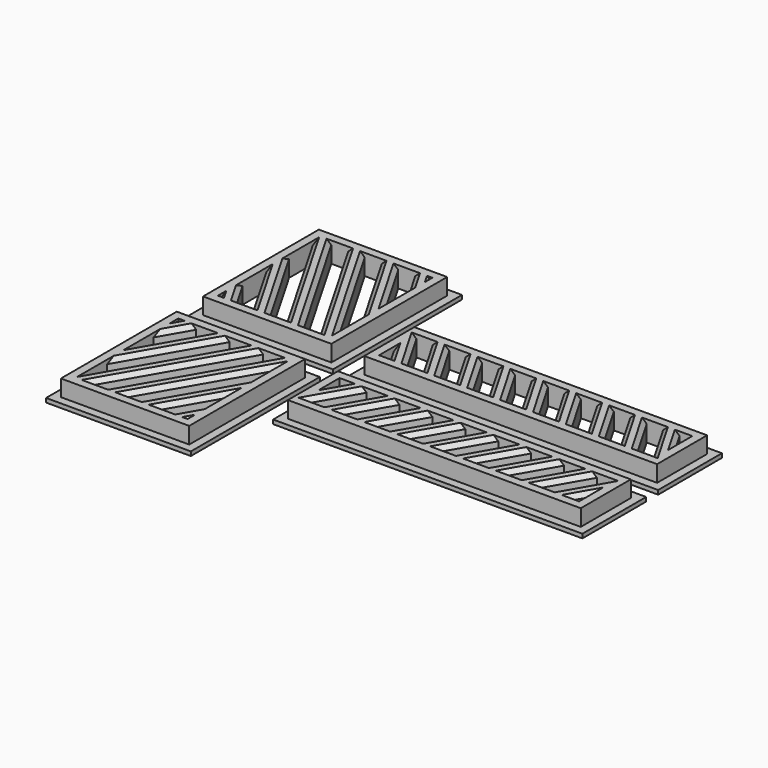
from build123d import *

# Parameters (mm, degrees)
F0_W      = 15.6
F0_H      = 17.6
F1_DEPTH  = 2.5
F2_W      = 35.7645684853
F2_H      = 21.2578142527
F3_DEPTH  = 10
F4_W      = 15.6
F4_H      = 17.6
F4_W_2    = 13.6
F4_H_2    = 15.6
F5_DEPTH  = 2.5
F6_W      = 17.6
F6_H      = 19.6
F6_W_2    = 15.6
F6_H_2    = 17.6
F7_DEPTH  = 0.5
F8_SIZE   = 0.5
F9_W      = 35.6
F9_H      = 7.6
F10_DEPTH = 2.5
F11_W     = 70.1136225462
F11_H     = 15.9944170155
F12_DEPTH = 25
F13_W     = 35.6
F13_H     = 7.6
F13_W_2   = 33.6
F13_H_2   = 5.6
F14_DEPTH = 2.5
F15_W     = 37.6
F15_H     = 9.6891392594
F15_W_2   = 35.6
F15_H_2   = 7.6
F16_DEPTH = 0.5
F17_SIZE  = 0.5


with BuildPart() as f1:
    # F0 (on Top) → F1 (new body)
    with BuildSketch(Plane.XY):
        with Locations((-9.8, 8.8)):
            Rectangle(F0_W, F0_H)
    extrude(amount=F1_DEPTH)

    # F2 (on Top) → F3 (cut)
    with BuildSketch(Plane.XY):
        with Locations((-9.857636116, 8.6271929322)):
            Rectangle(F2_W, F2_H)
        Polygon((-13.85, 0), (-15.85, 0), (-26.0113647377, 17.6), (-24.0113647377, 17.6), align=None, mode=Mode.SUBTRACT)
        Polygon((-21.940212315, 17.6), (-19.940212315, 17.6), (-9.7788475773, 0), (-11.7788475773, 0), align=None, mode=Mode.SUBTRACT)
        Polygon((-17.8690598923, 17.6), (-15.8690598923, 17.6), (-5.7076951546, 0), (-7.7076951546, 0), align=None, mode=Mode.SUBTRACT)
        Polygon((-13.7979074696, 17.6), (-11.7979074696, 17.6), (-1.6365427319, 0), (-3.6365427319, 0), align=None, mode=Mode.SUBTRACT)
        Polygon((-9.7267550469, 17.6), (-7.7267550469, 17.6), (2.4346096908, 0), (0.4346096908, 0), align=None, mode=Mode.SUBTRACT)
        Polygon((-5.6556026242, 17.6), (-3.6556026242, 17.6), (6.5057621135, 0), (4.5057621135, 0), align=None, mode=Mode.SUBTRACT)
    extrude(amount=F3_DEPTH, mode=Mode.SUBTRACT)

    # F4 (on Top) → F5 (join)
    with BuildSketch(Plane.XY):
        with Locations((-9.8, 8.8)):
            Rectangle(F4_W, F4_H)
        with Locations((-9.8, 8.8)):
            Rectangle(F4_W_2, F4_H_2, mode=Mode.SUBTRACT)
    extrude(amount=F5_DEPTH)

    # F6 (on face) → F7 (join)
    with BuildSketch(Plane(origin=(0, 0, 0), x_dir=(1, 0, 0), z_dir=(0, 0, -1))):
        with Locations((-9.8, -8.8)):
            Rectangle(F6_W, F6_H)
        with Locations((-9.8, -8.8)):
            Rectangle(F6_W_2, F6_H_2, mode=Mode.SUBTRACT)
    extrude(amount=-F7_DEPTH)

    # F8
    f8_edges = [f1.edges().sort_by_distance(p)[0] for p in [
        (-15.513675, 2.88157, 2.5),
        (-14.478099, 4.67524, 2.5),
        (-12.442523, 8.200962, 0),
        (-10.788378, 8.8, 2.5),
        (-8.717225, 8.8, 2.5),
        (-7.110279, 9.480789, 2.5),
        (-6.074702, 11.274459, 2.5),
        (-5.074702, 13.00651, 2.5),
        (-4.039126, 14.800181, 2.5),
        (-16.513675, 1.149519, 2.5),
        (-3.039126, 16.532231, 2.5),
        (-12.442523, 8.200962, 2.5),
        (-13.478099, 6.407291, 2.5),
    ]]
    chamfer(f8_edges, length=F8_SIZE)


with BuildPart() as f10:
    # F9 (on Top) → F10 (new body)
    with BuildSketch(Plane.XY):
        with Locations((19.8, 3.8)):
            Rectangle(F9_W, F9_H)
    extrude(amount=F10_DEPTH)

    # F11 (on Top) → F12 (cut)
    with BuildSketch(Plane.XY):
        with Locations((32.6393267076, 4.0027914923)):
            Rectangle(F11_W, F11_H)
        Polygon((6.8688021535, 0), (4.8688021535, 0), (0.25, 8), (2.25, 8), align=None, mode=Mode.SUBTRACT)
        Polygon((6.25, 8), (10.8688021535, 0), (8.8688021535, 0), (4.25, 8), align=None, mode=Mode.SUBTRACT)
        Polygon((10.25, 8), (14.8688021535, 0), (12.8688021535, 0), (8.25, 8), align=None, mode=Mode.SUBTRACT)
        Polygon((14.25, 8), (18.8688021535, 0), (16.8688021535, 0), (12.25, 8), align=None, mode=Mode.SUBTRACT)
        Polygon((18.25, 8), (22.8688021535, 0), (20.8688021535, 0), (16.25, 8), align=None, mode=Mode.SUBTRACT)
        Polygon((22.25, 8), (26.8688021535, 0), (24.8688021535, 0), (20.25, 8), align=None, mode=Mode.SUBTRACT)
        Polygon((26.25, 8), (30.8688021535, 0), (28.8688021535, 0), (24.25, 8), align=None, mode=Mode.SUBTRACT)
        Polygon((30.25, 8), (34.8688021535, 0), (32.8688021535, 0), (28.25, 8), align=None, mode=Mode.SUBTRACT)
        Polygon((34.25, 8), (38.8688021535, 0), (36.8688021535, 0), (32.25, 8), align=None, mode=Mode.SUBTRACT)
        Polygon((38.25, 8), (42.8688021535, 0), (40.8688021535, 0), (36.25, 8), align=None, mode=Mode.SUBTRACT)
        Polygon((42.25, 8), (46.8688021535, 0), (44.8688021535, 0), (40.25, 8), align=None, mode=Mode.SUBTRACT)
        Polygon((46.25, 8), (50.8688021535, 0), (48.8688021535, 0), (44.25, 8), align=None, mode=Mode.SUBTRACT)
        Polygon((50.25, 8), (54.8688021535, 0), (52.8688021535, 0), (48.25, 8), align=None, mode=Mode.SUBTRACT)
        Polygon((54.25, 8), (58.8688021535, 0), (56.8688021535, 0), (52.25, 8), align=None, mode=Mode.SUBTRACT)
        Polygon((58.25, 8), (62.8688021535, 0), (60.8688021535, 0), (56.25, 8), align=None, mode=Mode.SUBTRACT)
    extrude(amount=F12_DEPTH, mode=Mode.SUBTRACT)

    # F13 (on Top) → F14 (join)
    with BuildSketch(Plane.XY):
        with Locations((19.8, 3.8)):
            Rectangle(F13_W, F13_H)
        with Locations((19.8, 3.8)):
            Rectangle(F13_W_2, F13_H_2, mode=Mode.SUBTRACT)
    extrude(amount=F14_DEPTH)

    # F15 (on face) → F16 (join)
    with BuildSketch(Plane(origin=(0, 0, 0), x_dir=(1, 0, 0), z_dir=(0, 0, -1))):
        with Locations((19.8, -3.7554303703)):
            Rectangle(F15_W, F15_H)
        with Locations((19.8, -3.8)):
            Rectangle(F15_W_2, F15_H_2, mode=Mode.SUBTRACT)
    extrude(amount=-F16_DEPTH)

    # F17
    f17_edges = [f10.edges().sort_by_distance(p)[0] for p in [
        (8.674871, 3.8, 2.5),
        (10.674871, 3.8, 2.5),
        (12.674871, 3.8, 2.5),
        (14.674871, 3.8, 2.5),
        (16.674871, 3.8, 2.5),
        (18.674871, 3.8, 2.5),
        (20.674871, 3.8, 2.5),
        (22.674871, 3.8, 2.5),
        (24.674871, 3.8, 2.5),
        (26.674871, 3.8, 2.5),
        (28.674871, 3.8, 2.5),
        (30.674871, 3.8, 2.5),
        (32.674871, 3.8, 2.5),
        (34.674871, 3.8, 2.5),
        (35.829145, 5.26484, 2.5),
        (4.674871, 3.8, 2.5),
        (6.674871, 3.8, 2.5),
        (3.645726, 2.11843, 2.5),
    ]]
    chamfer(f17_edges, length=F17_SIZE)


with BuildPart() as f19_1:
    # F19: instance of F1
    add(f1.part.mirror(Plane(origin=(-9.8, -2, 0.25), x_dir=(1, 0, 0), z_dir=(0, -1, 0))))


with BuildPart() as f20_1:
    # F20: instance of F10
    add(f10.part.mirror(Plane(origin=(-9.8, -2, 0.25), x_dir=(1, 0, 0), z_dir=(0, -1, 0))))


solid = Compound([f1.part, f10.part, f19_1.part, f20_1.part])
